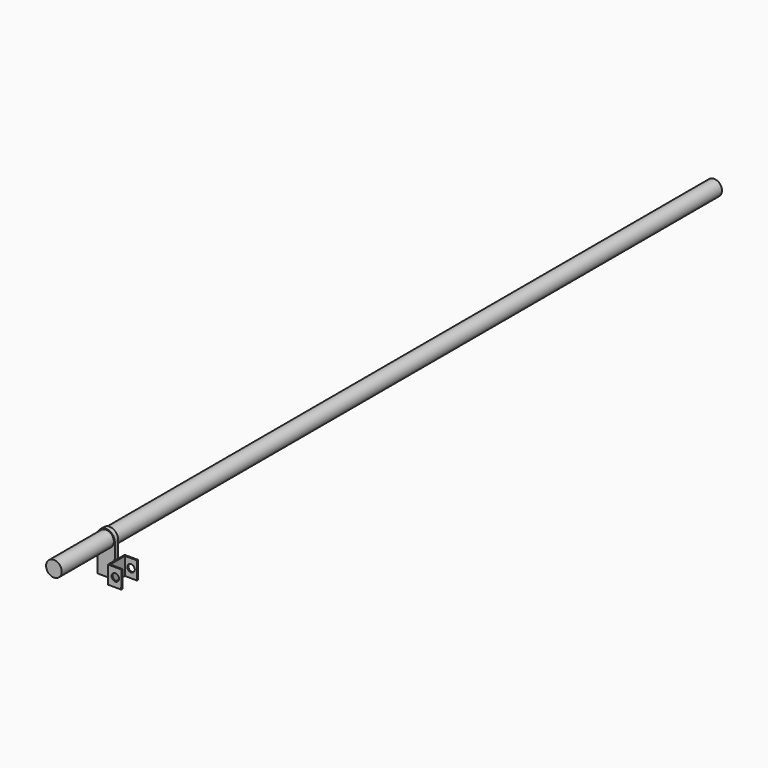
from build123d import *

# Parameters (mm, degrees)
F1_DEPTH      = 1.27
F2_R          = 2.2887754184
F3_DEPTH      = 220.98
F3_DEPTH_BACK = 20.32
F4_W          = 1.27
F4_H          = 3.4091206923
F5_DEPTH      = 3.937
F6_T          = -0.381
F7_R          = 1.080450049
F8_DEPTH      = 11.176


# Not quite as in the source:
# - a feature names something its author has since deleted; it is built from what else it names


with BuildPart() as f1:
    # F0 (on Front) → F1 (new body)
    with BuildSketch(Plane.XZ):
        with BuildLine():
            ThreePointArc((-2.5559609307, 5.4012401961), (0, 2.8452792654), (2.5559609307, 5.4012401961))
            ThreePointArc((2.5559609307, 5.4012401961), (0, 7.9572011268), (-2.5559609307, 5.4012401961))
        make_face()
        with BuildLine():
            Line((2.5559609307, 1.721014436), (2.5559609307, 5.4012401961))
            ThreePointArc((2.5559609307, 5.4012401961), (0, 2.8452792654), (-2.5559609307, 5.4012401961))
            Line((-2.5559609307, 5.4012401961), (-2.5559609307, 4.3758706689))
            Line((-2.5559609307, 4.3758706689), (-2.5559609307, -2.8266729787))
            Line((-2.5559609307, -2.8266729787), (-2.5559609307, -4.3681138195))
            Line((-2.5559609307, -4.3681138195), (2.5204877513, -4.3681138195))
            Line((2.5204877513, -4.3681138195), (2.5204877513, -2.8266729787))
            Line((2.5204877513, -2.8266729787), (2.5559609307, 1.721014436))
        make_face()
    extrude(amount=-F1_DEPTH)

    # F2 (on face) → F3 (join, two sides)
    with BuildSketch(Plane(origin=(0, 1.27, 0), x_dir=(-1, 0, 0), z_dir=(0, 1, 0))) as f3_sk:
        with Locations((0, 5.4012401961)):
            Circle(F2_R)
    extrude(amount=F3_DEPTH)
    extrude(f3_sk.sketch, amount=-F3_DEPTH_BACK)


with BuildPart() as f5:
    # F4 (on face) → F5 (new body)
    with BuildSketch(Plane(origin=(2.5423818682, 0, -0.0198312593), x_dir=(0, 1, 0), z_dir=(0.9999695793, 0, -0.0078000304))):
        Polygon((-2.497356755, -4.576918826), (3.6564493494, -4.576918826), (3.6564493494, 0.6021935842), (1.27, 0.6021935842), (1.27, -2.8069271081), (0, -2.8069271081), (0, 0.6021935842), (-2.497356755, 0.6021935842), align=None)
        with Locations((0.635, -1.102366762)):
            Rectangle(F4_W, F4_H)
    extrude(amount=F5_DEPTH)

    # F6
    f6_openings = [f5.faces().sort_by_distance(p)[0] for p in [
        (6.463761, 0.579546, -2.037842),
        (4.515519, 0.579546, 0.56699),
        (4.475122, 0.579546, -4.611965),
    ]]
    offset(amount=F6_T, openings=f6_openings)

    # F7 (on face) → F8 (cut)
    with BuildSketch(Plane.XZ.offset(2.497356755)):
        with Locations((4.7060133182, -2.0378421431)):
            Circle(F7_R)
    extrude(amount=-F8_DEPTH, mode=Mode.SUBTRACT)


solid = Compound([f1.part, f5.part])
